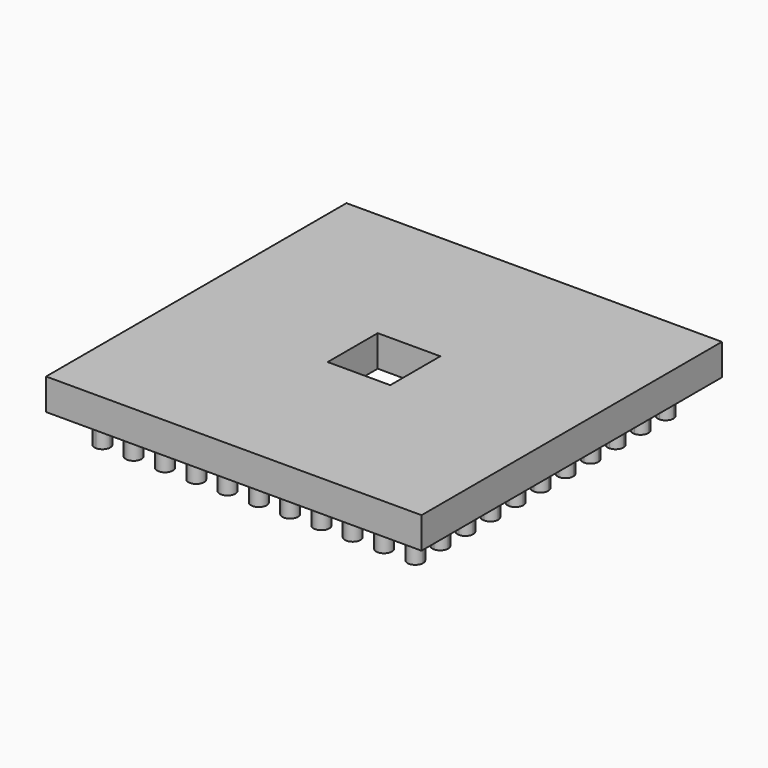
from build123d import *

# Parameters (mm, degrees)
F0_W     = 304.8
F0_H     = 304.8
F1_DEPTH = 25.4
F2_R     = 6.35
F3_DEPTH = 25.4
F5_DEPTH = 25.4


with BuildPart() as f1:
    # F0 (on Top) → F1 (new body)
    with BuildSketch(Plane.XY):
        with Locations((-18.4810393786, 92.4112985205)):
            Rectangle(F0_W, F0_H)
    extrude(amount=F1_DEPTH)

    # F2 (on face) → F3 (join)
    with BuildSketch(Plane(origin=(0, 0, 0), x_dir=(1, 0, 0), z_dir=(0, 0, -1))):
        with BuildLine():
            Line((-145.4810393786, 34.5887014795), (-145.4810393786, 40.9387014795))
            ThreePointArc((-145.4810393786, 40.9387014795), (-151.8310393786, 34.5887014795), (-145.4810393786, 28.2387014795))
            Line((-145.4810393786, 28.2387014795), (-145.4810393786, 34.5887014795))
        make_face()
        with BuildLine():
            Line((-145.4810393786, 9.1887014795), (-145.4810393786, 15.5387014795))
            ThreePointArc((-145.4810393786, 15.5387014795), (-151.8310393786, 9.1887014795), (-145.4810393786, 2.8387014795))
            Line((-145.4810393786, 2.8387014795), (-145.4810393786, 9.1887014795))
        make_face()
        with BuildLine():
            ThreePointArc((-139.1310393786, 9.1887014795), (-140.9909113181, 13.6788295401), (-145.4810393786, 15.5387014795))
            Line((-145.4810393786, 15.5387014795), (-145.4810393786, 9.1887014795))
            Line((-145.4810393786, 9.1887014795), (-145.4810393786, 2.8387014795))
            ThreePointArc((-145.4810393786, 2.8387014795), (-140.9909113181, 4.698573419), (-139.1310393786, 9.1887014795))
        make_face()
        with BuildLine():
            ThreePointArc((-139.1310393786, 34.5887014795), (-140.9909113181, 39.0788295401), (-145.4810393786, 40.9387014795))
            Line((-145.4810393786, 40.9387014795), (-145.4810393786, 34.5887014795))
            Line((-145.4810393786, 34.5887014795), (-145.4810393786, 28.2387014795))
            ThreePointArc((-145.4810393786, 28.2387014795), (-140.9909113181, 30.098573419), (-139.1310393786, 34.5887014795))
        make_face()
        with BuildLine():
            Line((-145.4810393786, -16.2112985205), (-145.4810393786, -9.8612985205))
            ThreePointArc((-145.4810393786, -9.8612985205), (-151.8310393786, -16.2112985205), (-145.4810393786, -22.5612985205))
            Line((-145.4810393786, -22.5612985205), (-145.4810393786, -16.2112985205))
        make_face()
        with BuildLine():
            ThreePointArc((-139.1310393786, -16.2112985205), (-140.9909113181, -11.7211704599), (-145.4810393786, -9.8612985205))
            Line((-145.4810393786, -9.8612985205), (-145.4810393786, -16.2112985205))
            Line((-145.4810393786, -16.2112985205), (-145.4810393786, -22.5612985205))
            ThreePointArc((-145.4810393786, -22.5612985205), (-140.9909113181, -20.701426581), (-139.1310393786, -16.2112985205))
        make_face()
        with BuildLine():
            Line((-145.4810393786, -41.6112985205), (-145.4810393786, -35.2612985205))
            ThreePointArc((-145.4810393786, -35.2612985205), (-151.8310393786, -41.6112985205), (-145.4810393786, -47.9612985205))
            Line((-145.4810393786, -47.9612985205), (-145.4810393786, -41.6112985205))
        make_face()
        with BuildLine():
            ThreePointArc((-139.1310393786, -41.6112985205), (-140.9909113181, -37.1211704599), (-145.4810393786, -35.2612985205))
            Line((-145.4810393786, -35.2612985205), (-145.4810393786, -41.6112985205))
            Line((-145.4810393786, -41.6112985205), (-145.4810393786, -47.9612985205))
            ThreePointArc((-145.4810393786, -47.9612985205), (-140.9909113181, -46.101426581), (-139.1310393786, -41.6112985205))
        make_face()
        with BuildLine():
            Line((-145.4810393786, -67.0112985205), (-145.4810393786, -60.6612985205))
            ThreePointArc((-145.4810393786, -60.6612985205), (-151.8310393786, -67.0112985205), (-145.4810393786, -73.3612985205))
            Line((-145.4810393786, -73.3612985205), (-145.4810393786, -67.0112985205))
        make_face()
        with BuildLine():
            ThreePointArc((-139.1310393786, -67.0112985205), (-140.9909113181, -62.5211704599), (-145.4810393786, -60.6612985205))
            Line((-145.4810393786, -60.6612985205), (-145.4810393786, -67.0112985205))
            Line((-145.4810393786, -67.0112985205), (-145.4810393786, -73.3612985205))
            ThreePointArc((-145.4810393786, -73.3612985205), (-140.9909113181, -71.501426581), (-139.1310393786, -67.0112985205))
        make_face()
        with BuildLine():
            ThreePointArc((-139.1310393786, -92.4112985205), (-140.9909113181, -87.9211704599), (-145.4810393786, -86.0612985205))
            Line((-145.4810393786, -86.0612985205), (-145.4810393786, -92.4112985205))
            Line((-145.4810393786, -92.4112985205), (-145.4810393786, -98.7612985205))
            ThreePointArc((-145.4810393786, -98.7612985205), (-140.9909113181, -96.901426581), (-139.1310393786, -92.4112985205))
        make_face()
        with BuildLine():
            Line((-145.4810393786, -92.4112985205), (-145.4810393786, -86.0612985205))
            ThreePointArc((-145.4810393786, -86.0612985205), (-151.8310393786, -92.4112985205), (-145.4810393786, -98.7612985205))
            Line((-145.4810393786, -98.7612985205), (-145.4810393786, -92.4112985205))
        make_face()
        with BuildLine():
            Line((-145.4810393786, -117.8112985205), (-145.4810393786, -124.1612985205))
            ThreePointArc((-145.4810393786, -124.1612985205), (-140.9909113181, -122.301426581), (-139.1310393786, -117.8112985205))
            ThreePointArc((-139.1310393786, -117.8112985205), (-140.9909113181, -113.3211704599), (-145.4810393786, -111.4612985205))
            Line((-145.4810393786, -111.4612985205), (-145.4810393786, -117.8112985205))
        make_face()
        with BuildLine():
            ThreePointArc((-145.4810393786, -111.4612985205), (-151.8310393786, -117.8112985205), (-145.4810393786, -124.1612985205))
            Line((-145.4810393786, -124.1612985205), (-145.4810393786, -117.8112985205))
            Line((-145.4810393786, -117.8112985205), (-145.4810393786, -111.4612985205))
        make_face()
        with BuildLine():
            ThreePointArc((-145.4810393786, -136.8612985205), (-151.8310393786, -143.2112985205), (-145.4810393786, -149.5612985205))
            Line((-145.4810393786, -149.5612985205), (-145.4810393786, -143.2112985205))
            Line((-145.4810393786, -143.2112985205), (-145.4810393786, -136.8612985205))
        make_face()
        with BuildLine():
            Line((-145.4810393786, -143.2112985205), (-145.4810393786, -149.5612985205))
            ThreePointArc((-145.4810393786, -149.5612985205), (-140.9909113181, -147.701426581), (-139.1310393786, -143.2112985205))
            ThreePointArc((-139.1310393786, -143.2112985205), (-140.9909113181, -138.7211704599), (-145.4810393786, -136.8612985205))
            Line((-145.4810393786, -136.8612985205), (-145.4810393786, -143.2112985205))
        make_face()
        with Locations((-120.0810393786, 34.5887014795)):
            Circle(F2_R)
        with BuildLine():
            ThreePointArc((-101.0310393786, 34.5887014795), (-94.6810393786, 28.2387014795), (-88.3310393786, 34.5887014795))
            Line((-88.3310393786, 34.5887014795), (-94.6810393786, 34.5887014795))
            Line((-94.6810393786, 34.5887014795), (-101.0310393786, 34.5887014795))
        make_face()
        with BuildLine():
            Line((-94.6810393786, 34.5887014795), (-88.3310393786, 34.5887014795))
            ThreePointArc((-88.3310393786, 34.5887014795), (-94.6810393786, 40.9387014795), (-101.0310393786, 34.5887014795))
            Line((-101.0310393786, 34.5887014795), (-94.6810393786, 34.5887014795))
        make_face()
        with BuildLine():
            Line((-69.2810393786, 34.5887014795), (-62.9310393786, 34.5887014795))
            ThreePointArc((-62.9310393786, 34.5887014795), (-69.2810393786, 40.9387014795), (-75.6310393786, 34.5887014795))
            Line((-75.6310393786, 34.5887014795), (-69.2810393786, 34.5887014795))
        make_face()
        with BuildLine():
            ThreePointArc((-75.6310393786, 34.5887014795), (-69.2810393786, 28.2387014795), (-62.9310393786, 34.5887014795))
            Line((-62.9310393786, 34.5887014795), (-69.2810393786, 34.5887014795))
            Line((-69.2810393786, 34.5887014795), (-75.6310393786, 34.5887014795))
        make_face()
        with BuildLine():
            Line((-43.8810393786, 34.5887014795), (-37.5310393786, 34.5887014795))
            ThreePointArc((-37.5310393786, 34.5887014795), (-43.8810393786, 40.9387014795), (-50.2310393786, 34.5887014795))
            Line((-50.2310393786, 34.5887014795), (-43.8810393786, 34.5887014795))
        make_face()
        with BuildLine():
            ThreePointArc((-50.2310393786, 34.5887014795), (-43.8810393786, 28.2387014795), (-37.5310393786, 34.5887014795))
            Line((-37.5310393786, 34.5887014795), (-43.8810393786, 34.5887014795))
            Line((-43.8810393786, 34.5887014795), (-50.2310393786, 34.5887014795))
        make_face()
        with BuildLine():
            Line((-18.4810393786, 34.5887014795), (-12.1310393786, 34.5887014795))
            ThreePointArc((-12.1310393786, 34.5887014795), (-18.4810393786, 40.9387014795), (-24.8310393786, 34.5887014795))
            Line((-24.8310393786, 34.5887014795), (-18.4810393786, 34.5887014795))
        make_face()
        with BuildLine():
            ThreePointArc((-24.8310393786, 34.5887014795), (-18.4810393786, 28.2387014795), (-12.1310393786, 34.5887014795))
            Line((-12.1310393786, 34.5887014795), (-18.4810393786, 34.5887014795))
            Line((-18.4810393786, 34.5887014795), (-24.8310393786, 34.5887014795))
        make_face()
        with BuildLine():
            Line((6.9189606214, 34.5887014795), (13.2689606214, 34.5887014795))
            ThreePointArc((13.2689606214, 34.5887014795), (6.9189606214, 40.9387014795), (0.5689606214, 34.5887014795))
            Line((0.5689606214, 34.5887014795), (6.9189606214, 34.5887014795))
        make_face()
        with BuildLine():
            ThreePointArc((0.5689606214, 34.5887014795), (6.9189606214, 28.2387014795), (13.2689606214, 34.5887014795))
            Line((13.2689606214, 34.5887014795), (6.9189606214, 34.5887014795))
            Line((6.9189606214, 34.5887014795), (0.5689606214, 34.5887014795))
        make_face()
        with BuildLine():
            Line((32.3189606214, 34.5887014795), (38.6689606214, 34.5887014795))
            ThreePointArc((38.6689606214, 34.5887014795), (32.3189606214, 40.9387014795), (25.9689606214, 34.5887014795))
            Line((25.9689606214, 34.5887014795), (32.3189606214, 34.5887014795))
        make_face()
        with BuildLine():
            ThreePointArc((25.9689606214, 34.5887014795), (32.3189606214, 28.2387014795), (38.6689606214, 34.5887014795))
            Line((38.6689606214, 34.5887014795), (32.3189606214, 34.5887014795))
            Line((32.3189606214, 34.5887014795), (25.9689606214, 34.5887014795))
        make_face()
        with BuildLine():
            Line((57.7189606214, 34.5887014795), (64.0689606214, 34.5887014795))
            ThreePointArc((64.0689606214, 34.5887014795), (57.7189606214, 40.9387014795), (51.3689606214, 34.5887014795))
            Line((51.3689606214, 34.5887014795), (57.7189606214, 34.5887014795))
        make_face()
        with BuildLine():
            ThreePointArc((51.3689606214, 34.5887014795), (57.7189606214, 28.2387014795), (64.0689606214, 34.5887014795))
            Line((64.0689606214, 34.5887014795), (57.7189606214, 34.5887014795))
            Line((57.7189606214, 34.5887014795), (51.3689606214, 34.5887014795))
        make_face()
        with BuildLine():
            Line((83.1189606214, 34.5887014795), (89.4689606214, 34.5887014795))
            ThreePointArc((89.4689606214, 34.5887014795), (83.1189606214, 40.9387014795), (76.7689606214, 34.5887014795))
            Line((76.7689606214, 34.5887014795), (83.1189606214, 34.5887014795))
        make_face()
        with BuildLine():
            ThreePointArc((76.7689606214, 34.5887014795), (83.1189606214, 28.2387014795), (89.4689606214, 34.5887014795))
            Line((89.4689606214, 34.5887014795), (83.1189606214, 34.5887014795))
            Line((83.1189606214, 34.5887014795), (76.7689606214, 34.5887014795))
        make_face()
        with BuildLine():
            Line((108.5189606214, 34.5887014795), (108.5189606214, 28.2387014795))
            ThreePointArc((108.5189606214, 28.2387014795), (113.0090886819, 30.098573419), (114.8689606214, 34.5887014795))
            ThreePointArc((114.8689606214, 34.5887014795), (108.5189606214, 40.9387014795), (102.1689606214, 34.5887014795))
            Line((102.1689606214, 34.5887014795), (108.5189606214, 34.5887014795))
        make_face()
        with BuildLine():
            ThreePointArc((102.1689606214, 34.5887014795), (104.0288325608, 30.098573419), (108.5189606214, 28.2387014795))
            Line((108.5189606214, 28.2387014795), (108.5189606214, 34.5887014795))
            Line((108.5189606214, 34.5887014795), (102.1689606214, 34.5887014795))
        make_face()
        with BuildLine():
            Line((108.5189606214, 9.1887014795), (108.5189606214, 2.8387014795))
            ThreePointArc((108.5189606214, 2.8387014795), (113.0090886819, 4.698573419), (114.8689606214, 9.1887014795))
            ThreePointArc((114.8689606214, 9.1887014795), (113.0090886819, 13.6788295401), (108.5189606214, 15.5387014795))
            Line((108.5189606214, 15.5387014795), (108.5189606214, 9.1887014795))
        make_face()
        with BuildLine():
            ThreePointArc((108.5189606214, 15.5387014795), (102.1689606214, 9.1887014795), (108.5189606214, 2.8387014795))
            Line((108.5189606214, 2.8387014795), (108.5189606214, 9.1887014795))
            Line((108.5189606214, 9.1887014795), (108.5189606214, 15.5387014795))
        make_face()
        with BuildLine():
            Line((108.5189606214, -16.2112985205), (108.5189606214, -22.5612985205))
            ThreePointArc((108.5189606214, -22.5612985205), (113.0090886819, -20.701426581), (114.8689606214, -16.2112985205))
            ThreePointArc((114.8689606214, -16.2112985205), (113.0090886819, -11.7211704599), (108.5189606214, -9.8612985205))
            Line((108.5189606214, -9.8612985205), (108.5189606214, -16.2112985205))
        make_face()
        with BuildLine():
            ThreePointArc((108.5189606214, -9.8612985205), (102.1689606214, -16.2112985205), (108.5189606214, -22.5612985205))
            Line((108.5189606214, -22.5612985205), (108.5189606214, -16.2112985205))
            Line((108.5189606214, -16.2112985205), (108.5189606214, -9.8612985205))
        make_face()
        with BuildLine():
            Line((108.5189606214, -41.6112985205), (108.5189606214, -47.9612985205))
            ThreePointArc((108.5189606214, -47.9612985205), (113.0090886819, -46.101426581), (114.8689606214, -41.6112985205))
            ThreePointArc((114.8689606214, -41.6112985205), (113.0090886819, -37.1211704599), (108.5189606214, -35.2612985205))
            Line((108.5189606214, -35.2612985205), (108.5189606214, -41.6112985205))
        make_face()
        with BuildLine():
            ThreePointArc((108.5189606214, -35.2612985205), (102.1689606214, -41.6112985205), (108.5189606214, -47.9612985205))
            Line((108.5189606214, -47.9612985205), (108.5189606214, -41.6112985205))
            Line((108.5189606214, -41.6112985205), (108.5189606214, -35.2612985205))
        make_face()
        with BuildLine():
            Line((108.5189606214, -67.0112985205), (108.5189606214, -73.3612985205))
            ThreePointArc((108.5189606214, -73.3612985205), (113.0090886819, -71.501426581), (114.8689606214, -67.0112985205))
            ThreePointArc((114.8689606214, -67.0112985205), (113.0090886819, -62.5211704599), (108.5189606214, -60.6612985205))
            Line((108.5189606214, -60.6612985205), (108.5189606214, -67.0112985205))
        make_face()
        with BuildLine():
            ThreePointArc((108.5189606214, -60.6612985205), (102.1689606214, -67.0112985205), (108.5189606214, -73.3612985205))
            Line((108.5189606214, -73.3612985205), (108.5189606214, -67.0112985205))
            Line((108.5189606214, -67.0112985205), (108.5189606214, -60.6612985205))
        make_face()
        with BuildLine():
            ThreePointArc((108.5189606214, -86.0612985205), (102.1689606214, -92.4112985205), (108.5189606214, -98.7612985205))
            Line((108.5189606214, -98.7612985205), (108.5189606214, -92.4112985205))
            Line((108.5189606214, -92.4112985205), (108.5189606214, -86.0612985205))
        make_face()
        with BuildLine():
            Line((108.5189606214, -92.4112985205), (108.5189606214, -98.7612985205))
            ThreePointArc((108.5189606214, -98.7612985205), (113.0090886819, -96.901426581), (114.8689606214, -92.4112985205))
            ThreePointArc((114.8689606214, -92.4112985205), (113.0090886819, -87.9211704599), (108.5189606214, -86.0612985205))
            Line((108.5189606214, -86.0612985205), (108.5189606214, -92.4112985205))
        make_face()
        with BuildLine():
            Line((108.5189606214, -117.8112985205), (108.5189606214, -124.1612985205))
            ThreePointArc((108.5189606214, -124.1612985205), (113.0090886819, -122.301426581), (114.8689606214, -117.8112985205))
            ThreePointArc((114.8689606214, -117.8112985205), (113.0090886819, -113.3211704599), (108.5189606214, -111.4612985205))
            Line((108.5189606214, -111.4612985205), (108.5189606214, -117.8112985205))
        make_face()
        with BuildLine():
            ThreePointArc((108.5189606214, -111.4612985205), (102.1689606214, -117.8112985205), (108.5189606214, -124.1612985205))
            Line((108.5189606214, -124.1612985205), (108.5189606214, -117.8112985205))
            Line((108.5189606214, -117.8112985205), (108.5189606214, -111.4612985205))
        make_face()
        with BuildLine():
            Line((108.5189606214, -143.2112985205), (108.5189606214, -149.5612985205))
            ThreePointArc((108.5189606214, -149.5612985205), (113.0090886819, -147.701426581), (114.8689606214, -143.2112985205))
            ThreePointArc((114.8689606214, -143.2112985205), (113.0090886819, -138.7211704599), (108.5189606214, -136.8612985205))
            Line((108.5189606214, -136.8612985205), (108.5189606214, -143.2112985205))
        make_face()
        with BuildLine():
            ThreePointArc((108.5189606214, -136.8612985205), (102.1689606214, -143.2112985205), (108.5189606214, -149.5612985205))
            Line((108.5189606214, -149.5612985205), (108.5189606214, -143.2112985205))
            Line((108.5189606214, -143.2112985205), (108.5189606214, -136.8612985205))
        make_face()
        with BuildLine():
            Line((108.5189606214, -168.6112985205), (108.5189606214, -174.9612985205))
            ThreePointArc((108.5189606214, -174.9612985205), (113.0090886819, -173.101426581), (114.8689606214, -168.6112985205))
            ThreePointArc((114.8689606214, -168.6112985205), (113.0090886819, -164.1211704599), (108.5189606214, -162.2612985205))
            Line((108.5189606214, -162.2612985205), (108.5189606214, -168.6112985205))
        make_face()
        with BuildLine():
            ThreePointArc((108.5189606214, -162.2612985205), (102.1689606214, -168.6112985205), (108.5189606214, -174.9612985205))
            Line((108.5189606214, -174.9612985205), (108.5189606214, -168.6112985205))
            Line((108.5189606214, -168.6112985205), (108.5189606214, -162.2612985205))
        make_face()
        with BuildLine():
            Line((108.5189606214, -194.0112985205), (108.5189606214, -200.3612985205))
            ThreePointArc((108.5189606214, -200.3612985205), (113.0090886819, -198.501426581), (114.8689606214, -194.0112985205))
            ThreePointArc((114.8689606214, -194.0112985205), (113.0090886819, -189.5211704599), (108.5189606214, -187.6612985205))
            Line((108.5189606214, -187.6612985205), (108.5189606214, -194.0112985205))
        make_face()
        with BuildLine():
            ThreePointArc((108.5189606214, -187.6612985205), (102.1689606214, -194.0112985205), (108.5189606214, -200.3612985205))
            Line((108.5189606214, -200.3612985205), (108.5189606214, -194.0112985205))
            Line((108.5189606214, -194.0112985205), (108.5189606214, -187.6612985205))
        make_face()
        with BuildLine():
            Line((108.5189606214, -219.4112985205), (102.1689606214, -219.4112985205))
            ThreePointArc((102.1689606214, -219.4112985205), (108.5189606214, -225.7612985205), (114.8689606214, -219.4112985205))
            ThreePointArc((114.8689606214, -219.4112985205), (113.0090886819, -214.9211704599), (108.5189606214, -213.0612985205))
            Line((108.5189606214, -213.0612985205), (108.5189606214, -219.4112985205))
        make_face()
        with BuildLine():
            ThreePointArc((108.5189606214, -213.0612985205), (104.0288325608, -214.9211704599), (102.1689606214, -219.4112985205))
            Line((102.1689606214, -219.4112985205), (108.5189606214, -219.4112985205))
            Line((108.5189606214, -219.4112985205), (108.5189606214, -213.0612985205))
        make_face()
        with BuildLine():
            ThreePointArc((89.4689606214, -219.4112985205), (83.1189606214, -213.0612985205), (76.7689606214, -219.4112985205))
            Line((76.7689606214, -219.4112985205), (83.1189606214, -219.4112985205))
            Line((83.1189606214, -219.4112985205), (89.4689606214, -219.4112985205))
        make_face()
        with BuildLine():
            Line((83.1189606214, -219.4112985205), (76.7689606214, -219.4112985205))
            ThreePointArc((76.7689606214, -219.4112985205), (83.1189606214, -225.7612985205), (89.4689606214, -219.4112985205))
            Line((89.4689606214, -219.4112985205), (83.1189606214, -219.4112985205))
        make_face()
        with BuildLine():
            ThreePointArc((64.0689606214, -219.4112985205), (57.7189606214, -213.0612985205), (51.3689606214, -219.4112985205))
            Line((51.3689606214, -219.4112985205), (57.7189606214, -219.4112985205))
            Line((57.7189606214, -219.4112985205), (64.0689606214, -219.4112985205))
        make_face()
        with BuildLine():
            Line((57.7189606214, -219.4112985205), (51.3689606214, -219.4112985205))
            ThreePointArc((51.3689606214, -219.4112985205), (57.7189606214, -225.7612985205), (64.0689606214, -219.4112985205))
            Line((64.0689606214, -219.4112985205), (57.7189606214, -219.4112985205))
        make_face()
        with BuildLine():
            ThreePointArc((38.6689606214, -219.4112985205), (32.3189606214, -213.0612985205), (25.9689606214, -219.4112985205))
            Line((25.9689606214, -219.4112985205), (32.3189606214, -219.4112985205))
            Line((32.3189606214, -219.4112985205), (38.6689606214, -219.4112985205))
        make_face()
        with BuildLine():
            Line((32.3189606214, -219.4112985205), (25.9689606214, -219.4112985205))
            ThreePointArc((25.9689606214, -219.4112985205), (32.3189606214, -225.7612985205), (38.6689606214, -219.4112985205))
            Line((38.6689606214, -219.4112985205), (32.3189606214, -219.4112985205))
        make_face()
        with BuildLine():
            ThreePointArc((13.2689606214, -219.4112985205), (6.9189606214, -213.0612985205), (0.5689606214, -219.4112985205))
            Line((0.5689606214, -219.4112985205), (6.9189606214, -219.4112985205))
            Line((6.9189606214, -219.4112985205), (13.2689606214, -219.4112985205))
        make_face()
        with BuildLine():
            Line((6.9189606214, -219.4112985205), (0.5689606214, -219.4112985205))
            ThreePointArc((0.5689606214, -219.4112985205), (6.9189606214, -225.7612985205), (13.2689606214, -219.4112985205))
            Line((13.2689606214, -219.4112985205), (6.9189606214, -219.4112985205))
        make_face()
        with BuildLine():
            ThreePointArc((-12.1310393786, -219.4112985205), (-18.4810393786, -213.0612985205), (-24.8310393786, -219.4112985205))
            Line((-24.8310393786, -219.4112985205), (-18.4810393786, -219.4112985205))
            Line((-18.4810393786, -219.4112985205), (-12.1310393786, -219.4112985205))
        make_face()
        with BuildLine():
            Line((-18.4810393786, -219.4112985205), (-24.8310393786, -219.4112985205))
            ThreePointArc((-24.8310393786, -219.4112985205), (-18.4810393786, -225.7612985205), (-12.1310393786, -219.4112985205))
            Line((-12.1310393786, -219.4112985205), (-18.4810393786, -219.4112985205))
        make_face()
        with BuildLine():
            ThreePointArc((-37.5310393786, -219.4112985205), (-43.8810393786, -213.0612985205), (-50.2310393786, -219.4112985205))
            Line((-50.2310393786, -219.4112985205), (-43.8810393786, -219.4112985205))
            Line((-43.8810393786, -219.4112985205), (-37.5310393786, -219.4112985205))
        make_face()
        with BuildLine():
            Line((-43.8810393786, -219.4112985205), (-50.2310393786, -219.4112985205))
            ThreePointArc((-50.2310393786, -219.4112985205), (-43.8810393786, -225.7612985205), (-37.5310393786, -219.4112985205))
            Line((-37.5310393786, -219.4112985205), (-43.8810393786, -219.4112985205))
        make_face()
        with BuildLine():
            ThreePointArc((-62.9310393786, -219.4112985205), (-69.2810393786, -213.0612985205), (-75.6310393786, -219.4112985205))
            Line((-75.6310393786, -219.4112985205), (-69.2810393786, -219.4112985205))
            Line((-69.2810393786, -219.4112985205), (-62.9310393786, -219.4112985205))
        make_face()
        with BuildLine():
            Line((-69.2810393786, -219.4112985205), (-75.6310393786, -219.4112985205))
            ThreePointArc((-75.6310393786, -219.4112985205), (-69.2810393786, -225.7612985205), (-62.9310393786, -219.4112985205))
            Line((-62.9310393786, -219.4112985205), (-69.2810393786, -219.4112985205))
        make_face()
        with BuildLine():
            ThreePointArc((-88.3310393786, -219.4112985205), (-94.6810393786, -213.0612985205), (-101.0310393786, -219.4112985205))
            Line((-101.0310393786, -219.4112985205), (-94.6810393786, -219.4112985205))
            Line((-94.6810393786, -219.4112985205), (-88.3310393786, -219.4112985205))
        make_face()
        with BuildLine():
            Line((-94.6810393786, -219.4112985205), (-101.0310393786, -219.4112985205))
            ThreePointArc((-101.0310393786, -219.4112985205), (-94.6810393786, -225.7612985205), (-88.3310393786, -219.4112985205))
            Line((-88.3310393786, -219.4112985205), (-94.6810393786, -219.4112985205))
        make_face()
        with BuildLine():
            ThreePointArc((-113.7310393786, -219.4112985205), (-120.0810393786, -213.0612985205), (-126.4310393786, -219.4112985205))
            Line((-126.4310393786, -219.4112985205), (-120.0810393786, -219.4112985205))
            Line((-120.0810393786, -219.4112985205), (-113.7310393786, -219.4112985205))
        make_face()
        with BuildLine():
            Line((-120.0810393786, -219.4112985205), (-126.4310393786, -219.4112985205))
            ThreePointArc((-126.4310393786, -219.4112985205), (-120.0810393786, -225.7612985205), (-113.7310393786, -219.4112985205))
            Line((-113.7310393786, -219.4112985205), (-120.0810393786, -219.4112985205))
        make_face()
        with BuildLine():
            Line((-145.4810393786, -219.4112985205), (-145.4810393786, -225.7612985205))
            ThreePointArc((-145.4810393786, -225.7612985205), (-140.9909113181, -223.901426581), (-139.1310393786, -219.4112985205))
            Line((-139.1310393786, -219.4112985205), (-145.4810393786, -219.4112985205))
        make_face()
        with BuildLine():
            ThreePointArc((-145.4810393786, -213.0612985205), (-151.8310393786, -219.4112985205), (-145.4810393786, -225.7612985205))
            Line((-145.4810393786, -225.7612985205), (-145.4810393786, -219.4112985205))
            Line((-145.4810393786, -219.4112985205), (-145.4810393786, -213.0612985205))
        make_face()
        with BuildLine():
            Line((-145.4810393786, -213.0612985205), (-145.4810393786, -219.4112985205))
            Line((-145.4810393786, -219.4112985205), (-139.1310393786, -219.4112985205))
            ThreePointArc((-139.1310393786, -219.4112985205), (-140.9909113181, -214.9211704599), (-145.4810393786, -213.0612985205))
        make_face()
        with BuildLine():
            Line((-145.4810393786, -194.0112985205), (-145.4810393786, -200.3612985205))
            ThreePointArc((-145.4810393786, -200.3612985205), (-140.9909113181, -198.501426581), (-139.1310393786, -194.0112985205))
            ThreePointArc((-139.1310393786, -194.0112985205), (-140.9909113181, -189.5211704599), (-145.4810393786, -187.6612985205))
            Line((-145.4810393786, -187.6612985205), (-145.4810393786, -194.0112985205))
        make_face()
        with BuildLine():
            ThreePointArc((-145.4810393786, -187.6612985205), (-151.8310393786, -194.0112985205), (-145.4810393786, -200.3612985205))
            Line((-145.4810393786, -200.3612985205), (-145.4810393786, -194.0112985205))
            Line((-145.4810393786, -194.0112985205), (-145.4810393786, -187.6612985205))
        make_face()
        with BuildLine():
            Line((-145.4810393786, -168.6112985205), (-145.4810393786, -174.9612985205))
            ThreePointArc((-145.4810393786, -174.9612985205), (-140.9909113181, -173.101426581), (-139.1310393786, -168.6112985205))
            ThreePointArc((-139.1310393786, -168.6112985205), (-140.9909113181, -164.1211704599), (-145.4810393786, -162.2612985205))
            Line((-145.4810393786, -162.2612985205), (-145.4810393786, -168.6112985205))
        make_face()
        with BuildLine():
            ThreePointArc((-145.4810393786, -162.2612985205), (-151.8310393786, -168.6112985205), (-145.4810393786, -174.9612985205))
            Line((-145.4810393786, -174.9612985205), (-145.4810393786, -168.6112985205))
            Line((-145.4810393786, -168.6112985205), (-145.4810393786, -162.2612985205))
        make_face()
    extrude(amount=F3_DEPTH)

    # F4 (on face) → F5 (cut)
    with BuildSketch(Plane(origin=(0, 0, 0), x_dir=(1, 0, 0), z_dir=(0, 0, -1))):
        Polygon((6.9189606214, -67.0112985205), (-18.4810393786, -67.0112985205), (-43.8810393786, -67.0112985205), (-43.8810393786, -117.8112985205), (6.9189606214, -117.8112985205), align=None)
    extrude(amount=-F5_DEPTH, mode=Mode.SUBTRACT)


solid = f1.part
